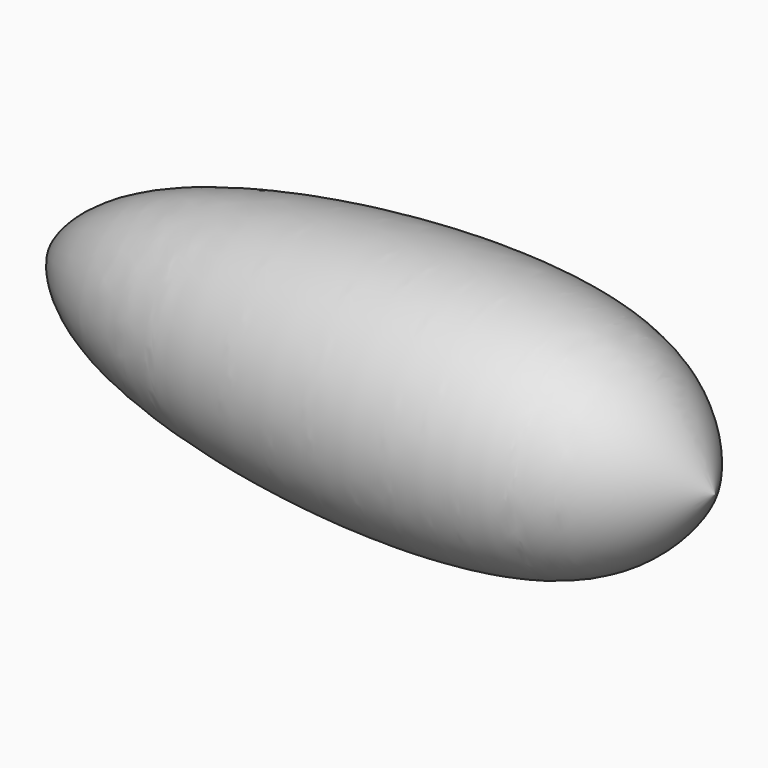
from build123d import *


with BuildPart() as f1:
    # F0 (on Front) → F1 (revolve)
    with BuildSketch(Plane.XZ):
        with BuildLine():
            add(Edge.make_bspline(
                [(-68.2042856836, 0), (-66.2853355341, 4.883688723), (-52.3310504766, 19.5485870419), (26.4070749094, 28.3755696825), (48.8389097154, 13.6340316385), (55.802586889, 0)],
                knots=[0, 0, 0, 0, 0.2371859218, 0.6806337043, 1, 1, 1, 1], degree=3))
            Line((-68.2042856836, 0), (-65.1125088334, 0))
            add(Edge.make_bspline(
                [(-65.1125088334, 0), (-61.9939343728, 3.737067747), (-53.6057089924, 15.4896776572), (33.7557618039, 24.9525646316), (44.2244058733, 7.0325665769), (51.2031279504, 0)],
                knots=[0, 0, 0, 0, 0.2274741313, 0.7115991588, 1, 1, 1, 1], degree=3))
            Line((51.2031279504, 0), (55.802586889, 0))
        make_face()
    revolve(axis=Axis((-6.2008493973, 0, 0), (1, 0, 0)))


solid = f1.part
